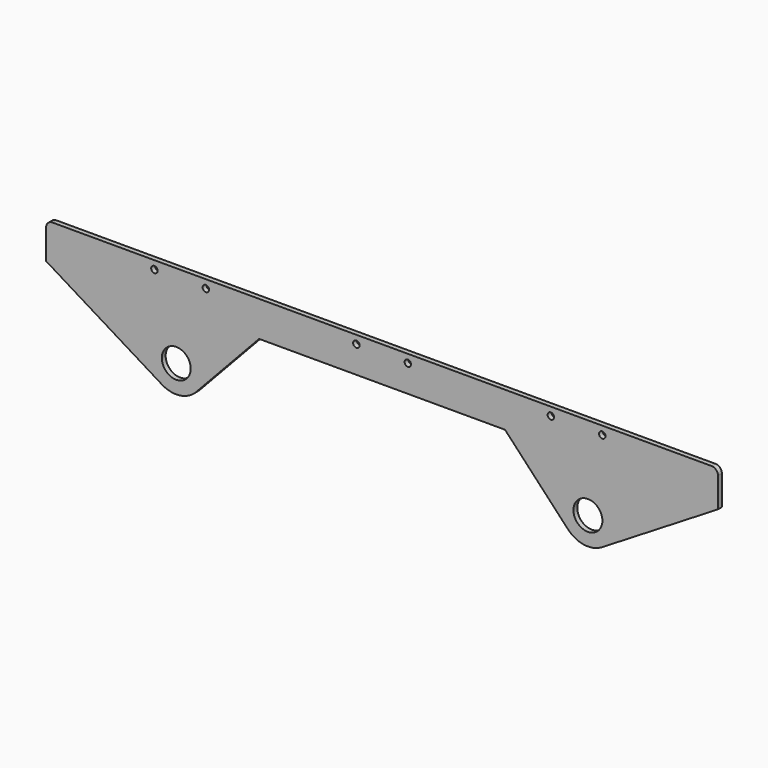
from build123d import *

# Parameters (mm, degrees)
F0_R     = 14.2875
F0_R_2   = 3.175
F1_DEPTH = 4.7625


# Not quite as in the source:
# - a feature names something its author has since deleted; it is built from what else it names


with BuildPart() as f1:
    # F0 (on Front) → F1 (new body)
    with BuildSketch(Plane.XZ):
        with BuildLine():
            Line((217.3001338382, 15.2277942336), (331.7059490892, 85.3303231618))
            Line((331.7059490892, 85.3303231618), (331.7059490892, 114.5403231618))
            ThreePointArc((331.7059490892, 114.5403231618), (329.8460771498, 119.0304512224), (325.3559490892, 120.8903231618))
            Line((325.3559490892, 120.8903231618), (0, 120.8903231618))
            Line((0, 120.8903231618), (-325.3559490892, 120.8903231618))
            ThreePointArc((-325.3559490892, 120.8903231618), (-329.8460771498, 119.0304512224), (-331.7059490892, 114.5403231618))
            Line((-331.7059490892, 114.5403231618), (-331.7059490892, 85.3303231618))
            Line((-331.7059490892, 85.3303231618), (-217.3001338382, 15.2277942336))
            ThreePointArc((-217.3001338382, 15.2277942336), (-199.5915875984, 11.4937311101), (-183.5057841229, 19.7872685874))
            Line((-183.5057841229, 19.7872685874), (-121.3841438293, 86.0923231618))
            Line((-121.3841438293, 86.0923231618), (0, 86.0923231618))
            Line((0, 86.0923231618), (121.3841438293, 86.0923231618))
            Line((121.3841438293, 86.0923231618), (183.5057841229, 19.7872685874))
            ThreePointArc((183.5057841229, 19.7872685874), (199.5915875984, 11.4937311101), (217.3001338382, 15.2277942336))
        make_face()
        with Locations((-203.2, 38.2389085481)):
            Circle(F0_R, mode=Mode.SUBTRACT)
        with Locations((203.2, 38.2389085481)):
            Circle(F0_R, mode=Mode.SUBTRACT)
        with Locations((-224.77598496, 112.7515938063)):
            Circle(F0_R_2, mode=Mode.SUBTRACT)
        with Locations((-173.97598496, 112.7515938063)):
            Circle(F0_R_2, mode=Mode.SUBTRACT)
        with Locations((-25.4, 112.7515938063)):
            Circle(F0_R_2, mode=Mode.SUBTRACT)
        with Locations((25.4, 112.7515938063)):
            Circle(F0_R_2, mode=Mode.SUBTRACT)
        with Locations((166.6059490892, 112.7515938063)):
            Circle(F0_R_2, mode=Mode.SUBTRACT)
        with Locations((217.4059490892, 112.7515938063)):
            Circle(F0_R_2, mode=Mode.SUBTRACT)
    extrude(amount=F1_DEPTH)


solid = f1.part
